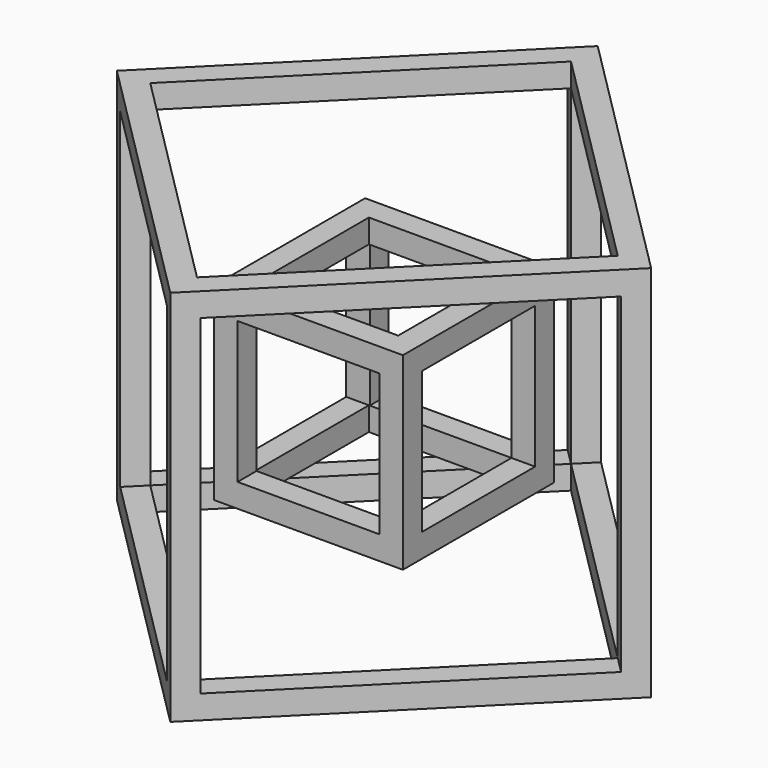
from build123d import *

# Parameters (mm, degrees)
F0_W      = 25.4
F0_H      = 25.4
F0_W_2    = 19.05
F0_H_2    = 19.05
F1_DEPTH  = 12.7
F2_W      = 19.05
F2_H      = 19.05
F3_DEPTH  = 25.4
F4_W      = 19.177
F4_H      = 19.05
F5_DEPTH  = 25.4
F7_W      = 50.8
F7_H      = 50.8
F7_W_2    = 44.45
F7_H_2    = 44.45
F8_DEPTH  = 25.4
F9_W      = 44.45
F9_H      = 44.45
F10_DEPTH = 76.201
F12_DEPTH = 50.801


with BuildPart() as f1:
    # F0 (on Front) → F1 (new body, symmetric)
    with BuildSketch(Plane.XZ):
        Rectangle(F0_W, F0_H)
        Rectangle(F0_W_2, F0_H_2, mode=Mode.SUBTRACT)
    extrude(amount=F1_DEPTH, both=True)

    # F2 (on face) → F3 (cut)
    with BuildSketch(Plane.YZ.offset(12.7)):
        Rectangle(F2_W, F2_H)
    extrude(amount=-F3_DEPTH, mode=Mode.SUBTRACT)

    # F4 (on face) → F5 (cut, through all)
    with BuildSketch(Plane.XY.offset(12.7)):
        with Locations((-0.0635, 0)):
            Rectangle(F4_W, F4_H)
    extrude(amount=-F5_DEPTH, mode=Mode.SUBTRACT)


with BuildPart() as f8:
    # F7 (on face) → F8 (new body, symmetric)
    with BuildSketch(Plane(origin=(0, 0, 0), x_dir=(0.7071067812, -0.7071067812, 0), z_dir=(-0.7071067812, -0.7071067812, 0))):
        Rectangle(F7_W, F7_H)
        Rectangle(F7_W_2, F7_H_2, mode=Mode.SUBTRACT)
    extrude(amount=F8_DEPTH, both=True)

    # F9 (on face) → F10 (cut, through all)
    with BuildSketch(Plane(origin=(-17.9605122421, 17.9605122421, 0), x_dir=(-0.7071067812, -0.7071067812, 0), z_dir=(-0.7071067812, 0.7071067812, 0))):
        Rectangle(F9_W, F9_H)
    extrude(amount=-F10_DEPTH, mode=Mode.SUBTRACT)

    # F11 (on face) → F12 (cut, through all)
    with BuildSketch(Plane.XY.offset(25.4)):
        Polygon((31.4308952947, 0), (0, 31.4308975528), (-31.430899811, 0), (0, -31.4309020691), align=None)
    extrude(amount=-F12_DEPTH, mode=Mode.SUBTRACT)


solid = Compound([f1.part, f8.part])
